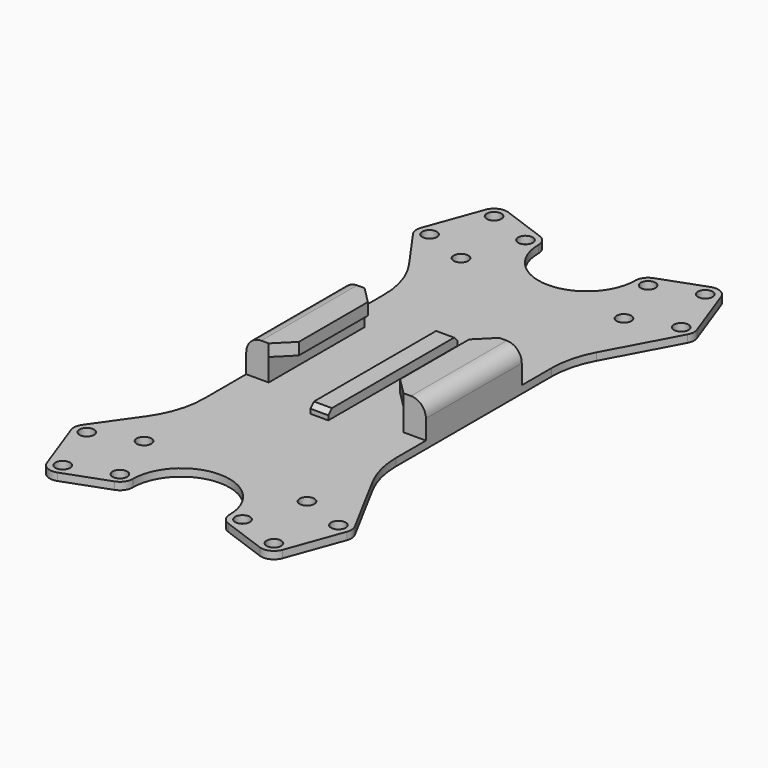
from build123d import *

# Parameters (mm, degrees)
F0_R     = 1.55
F1_DEPTH = 3.175
F2_W     = 3.81
F2_H     = 1.905
F3_DEPTH = 12.7
F5_SIZE  = 3.556
F6_DEPTH = 4.445
F7_DEPTH = 4.445
F8_SIZE  = 0.9525
F9_DEPTH = 1.5875
F10_R    = 3.175


# Not quite as in the source:
# - a feature names something its author has since deleted; it is built from what else it names


with BuildPart() as f1:
    # F0 (on Top) → F1 (new body)
    with BuildSketch(Plane.XY):
        with BuildLine():
            ThreePointArc((10.25, 53.7461577598), (0, 43.4961577598), (-10.25, 53.7461577598))
            ThreePointArc((-10.25, 53.7461577598), (-10.7473318782, 55.3234929598), (-12.0594446059, 56.330312467))
            Line((-12.0594446059, 56.330312467), (-21.4563708137, 59.7505139002))
            ThreePointArc((-21.4563708137, 59.7505139002), (-23.5591264276, 59.6587056074), (-24.981080915, 58.1069145872))
            Line((-24.981080915, 58.1069145872), (-29.2563327066, 46.3607568274))
            ThreePointArc((-29.2563327066, 46.3607568274), (-29.3979964883, 45.0563146846), (-28.9191151455, 43.8347130349))
            Line((-28.9191151455, 43.8347130349), (-22.5348535878, 34.7870060575))
            ThreePointArc((-22.5348535878, 34.7870060575), (-19.9421017302, 29.5652521638), (-19.05, 23.803895516))
            Line((-19.05, 23.803895516), (-19.05, 0))
            Line((-19.05, 0), (19.05, 0))
            Line((19.05, 0), (19.05, 20.6116865479))
            ThreePointArc((19.05, 20.6116865479), (19.6246909156, 25.2555485437), (21.3140896836, 29.6192231062))
            Line((21.3140896836, 29.6192231062), (29.095340906, 44.1199008802))
            ThreePointArc((29.095340906, 44.1199008802), (29.4151082328, 45.2231386646), (29.2563327066, 46.3607568274))
            Line((29.2563327066, 46.3607568274), (24.981080915, 58.1069145872))
            ThreePointArc((24.981080915, 58.1069145872), (23.5591264276, 59.6587056074), (21.4563708137, 59.7505139002))
            Line((21.4563708137, 59.7505139002), (12.0594446059, 56.330312467))
            ThreePointArc((12.0594446059, 56.330312467), (10.7473318782, 55.3234929598), (10.25, 53.7461577598))
        make_face()
        with Locations((-17.2752517916, 42)):
            Circle(F0_R, mode=Mode.SUBTRACT)
        with Locations((-26.6721779994, 45.4202014333)):
            Circle(F0_R, mode=Mode.SUBTRACT)
        with Locations((-22.3969262079, 57.1663591931)):
            Circle(F0_R, mode=Mode.SUBTRACT)
        with Locations((-13, 53.7461577598)):
            Circle(F0_R, mode=Mode.SUBTRACT)
        with Locations((17.2752517916, 42)):
            Circle(F0_R, mode=Mode.SUBTRACT)
        with Locations((13, 53.7461577598)):
            Circle(F0_R, mode=Mode.SUBTRACT)
        with Locations((26.6721779994, 45.4202014333)):
            Circle(F0_R, mode=Mode.SUBTRACT)
        with Locations((22.3969262079, 57.1663591931)):
            Circle(F0_R, mode=Mode.SUBTRACT)
    extrude(amount=F1_DEPTH)

    # F2 (on face) → F3 (join)
    with BuildSketch(Plane.XZ):
        Polygon((14.2875, 7.9375), (14.2875, 3.175), (19.05, 3.175), (19.05, 10.4775), (10.7315, 10.4775), (10.7315, 7.9375), align=None)
        with Locations((0, 4.1275)):
            Rectangle(F2_W, F2_H)
        Polygon((-19.05, 3.175), (-14.2875, 3.175), (-14.2875, 7.9375), (-10.7315, 7.9375), (-10.7315, 10.4775), (-19.05, 10.4775), align=None)
    extrude(amount=-F3_DEPTH)

    # F4: F1 across face


with BuildPart() as f1_1:
    add(f1.part)
    add(f1.part.mirror(Plane(origin=(0, 0, 3.9988214553), x_dir=(1, 0, 0), z_dir=(0, -1, 0))))

    # F5
    f5_edges = [f1_1.edges().sort_by_distance(p)[0] for p in [
        (10.7315, -12.7, 9.2075),
        (-10.7315, -12.7, 9.2075),
        (-10.7315, 12.7, 9.2075),
        (10.7315, 12.7, 9.2075),
    ]]
    chamfer(f5_edges, length=F5_SIZE)

    # F6 (add): a face of the model
    f6_faces = [f1_1.faces().sort_by_distance(p)[0] for p in [
        (0, -12.7, 4.1275),
    ]]
    extrude(f6_faces, amount=F6_DEPTH)

    # F7 (add): a face of the model
    f7_faces = [f1_1.faces().sort_by_distance(p)[0] for p in [
        (0, 12.7, 4.1275),
    ]]
    extrude(f7_faces, amount=F7_DEPTH)

    # F8
    f8_edges = [f1_1.edges().sort_by_distance(p)[0] for p in [
        (0, 17.145, 5.08),
        (0, -17.145, 5.08),
    ]]
    chamfer(f8_edges, length=F8_SIZE)

    # F9 (cut): a face of the model
    f9_faces = [f1_1.faces().sort_by_distance(p)[0] for p in [
        (0.1994717604, 0, 0),
    ]]
    extrude(f9_faces, amount=-F9_DEPTH, mode=Mode.SUBTRACT)

    # F10
    f10_edges = [f1_1.edges().sort_by_distance(p)[0] for p in [
        (-19.05, 0, 10.4775),
        (19.05, 0, 10.4775),
    ]]
    fillet(f10_edges, radius=F10_R)


solid = f1_1.part
